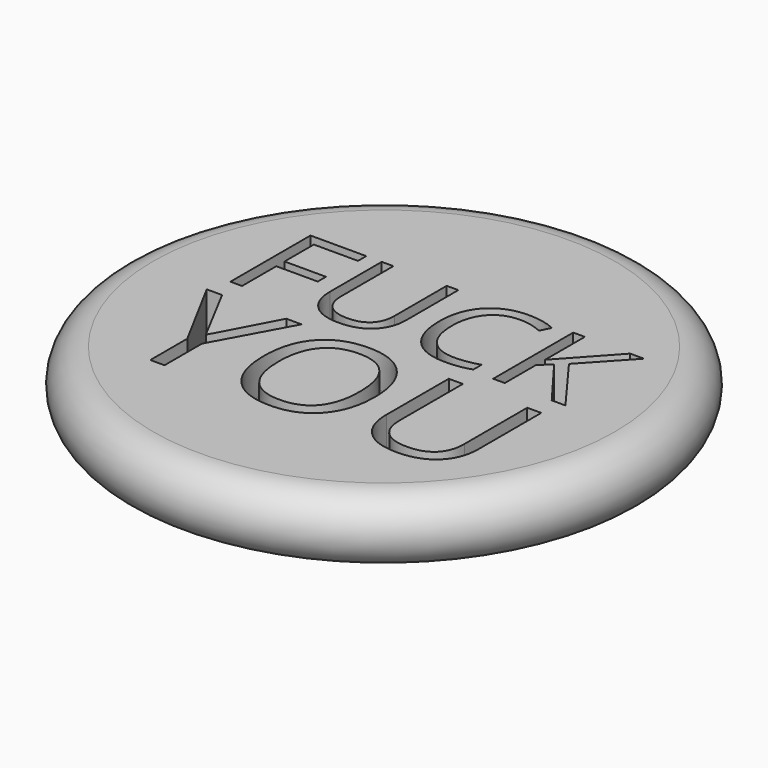
from build123d import *

# Parameters (mm, degrees)
F2_TEXT_SIZE   = 10.6205335922
F2_TEXT_SIZE_2 = 12.8317055189
F3_DEPTH       = 25
F4_DEPTH       = 25


# Not quite as in the source:
# - Text() gives the source's letters only with a copy of the font that has no kerning and outlines rounded to 1/6400 em; it was checked with that copy


with BuildPart() as f1:
    # F0 (on Front) → F1 (revolve)
    with BuildSketch(Plane.XZ):
        with BuildLine():
            Line((0, 2.5), (-17.5, 2.5))
            ThreePointArc((-17.5, 2.5), (-20, 0), (-17.5, -2.5))
            Line((-17.5, -2.5), (0, -2.5))
            Line((0, -2.5), (0, 2.5))
        make_face()
    revolve(axis=Axis((0, 0, 0), (0, 0, -1)))

    # F2 (on Top) → F3 (cut)
    with BuildSketch(Plane.XY):
        with Locations((-13.3314775303, 0.8123256266)):
            Text('FUCK', F2_TEXT_SIZE, font='Open Sans', text_align=(TextAlign.LEFT, TextAlign.BOTTOM))
        with Locations((-12.7722276375, -9.9886530079)):
            Text('YOU', F2_TEXT_SIZE_2, font='Open Sans', text_align=(TextAlign.LEFT, TextAlign.BOTTOM))
    extrude(amount=-F3_DEPTH, mode=Mode.SUBTRACT)

    # F2 (on Top) → F4 (cut)
    with BuildSketch(Plane.XY):
        with Locations((-13.3314775303, 0.8123256266)):
            Text('FUCK', F2_TEXT_SIZE, font='Open Sans', text_align=(TextAlign.LEFT, TextAlign.BOTTOM))
        with Locations((-12.7722276375, -9.9886530079)):
            Text('YOU', F2_TEXT_SIZE_2, font='Open Sans', text_align=(TextAlign.LEFT, TextAlign.BOTTOM))
    extrude(amount=F4_DEPTH, mode=Mode.SUBTRACT)


solid = f1.part
